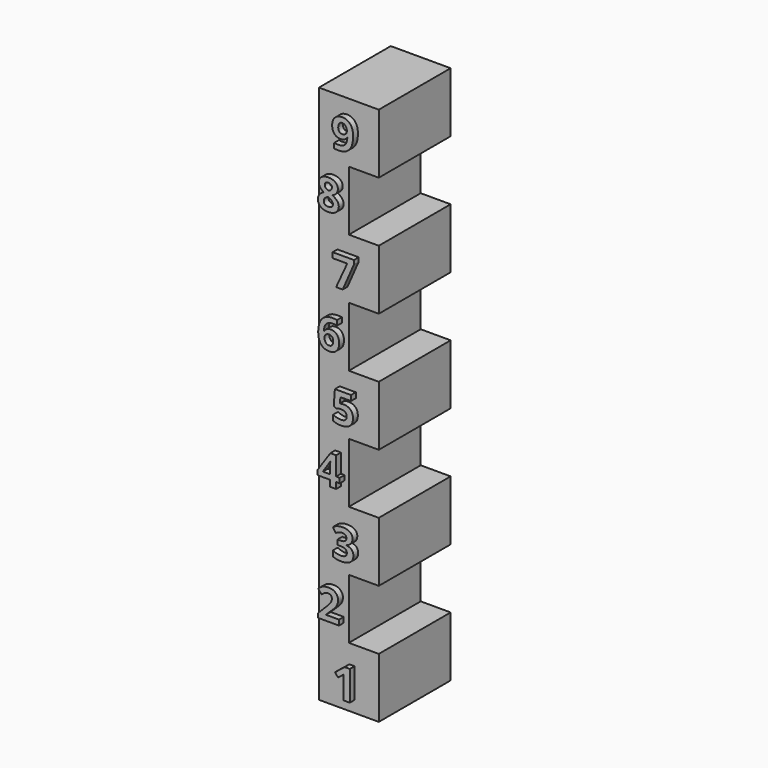
from build123d import *

# Parameters (mm, degrees)
F1_DEPTH     = 15
F2_TEXT_SIZE = 6.9444444444
F3_DEPTH     = 1
F4_TEXT_SIZE = 6.9444444444
F5_DEPTH     = 1


# Not quite as in the source:
# - Text() gives the source's letters only with a copy of the font that has no kerning and outlines rounded to 1/6400 em; it was checked with that copy


with BuildPart() as f1:
    # F0 (on Front) → F1 (new body)
    with BuildSketch(Plane.XZ):
        Polygon((17.6977999508, 53.6902362108), (17.6977999508, -36.3097637892), (22.6977999508, -36.3097637892), (27.6977999508, -36.3097637892), (27.6977999508, -26.3097637892), (22.6977999508, -26.3097637892), (22.6977999508, -16.3097637892), (27.6977999508, -16.3097637892), (27.6977999508, -6.3097637892), (22.6977999508, -6.3097637892), (22.6977999508, 3.6902362108), (27.6977999508, 3.6902362108), (27.6977999508, 13.6902362108), (22.6977999508, 13.6902362108), (22.6977999508, 23.6902362108), (27.6977999508, 23.6902362108), (27.6977999508, 33.6902362108), (22.6977999508, 33.6902362108), (22.6977999508, 43.6902362108), (27.6977999508, 43.6902362108), (27.6977999508, 53.6902362108), align=None)
    extrude(amount=F1_DEPTH)

    # F2 (on face) → F3 (join)
    with BuildSketch(Plane.XZ.offset(15)):
        with Locations((20.7831069488, -34.3956333771)):
            Text('1', F2_TEXT_SIZE, font='Open Sans', font_style=FontStyle.BOLD, text_align=(TextAlign.LEFT, TextAlign.BOTTOM))
        with Locations((18.1024699361, -23.6452650814)):
            Text('2', F2_TEXT_SIZE, font='Open Sans', font_style=FontStyle.BOLD, text_align=(TextAlign.LEFT, TextAlign.BOTTOM))
        with Locations((20.5617107408, -14.0193967335)):
            Text('3', F2_TEXT_SIZE, font='Open Sans', font_style=FontStyle.BOLD, text_align=(TextAlign.LEFT, TextAlign.BOTTOM))
        with Locations((18.1209300458, -3.7207709346)):
            Text('4', F2_TEXT_SIZE, font='Open Sans', font_style=FontStyle.BOLD, text_align=(TextAlign.LEFT, TextAlign.BOTTOM))
        with Locations((20.5431034747, 5.9468481503)):
            Text('5', F2_TEXT_SIZE, font='Open Sans', font_style=FontStyle.BOLD, text_align=(TextAlign.LEFT, TextAlign.BOTTOM))
        with Locations((18.136892487, 16.2113205343)):
            Text('6', F2_TEXT_SIZE, font='Open Sans', font_style=FontStyle.BOLD, text_align=(TextAlign.LEFT, TextAlign.BOTTOM))
        with Locations((20.6009032494, 25.9541989118)):
            Text('7', F2_TEXT_SIZE, font='Open Sans', font_style=FontStyle.BOLD, text_align=(TextAlign.LEFT, TextAlign.BOTTOM))
        with Locations((18.0933616431, 36.6414812207)):
            Text('8', F2_TEXT_SIZE, font='Open Sans', font_style=FontStyle.BOLD, text_align=(TextAlign.LEFT, TextAlign.BOTTOM))
        with Locations((20.4888266866, 46.2495227158)):
            Text('9', F2_TEXT_SIZE, font='Open Sans', font_style=FontStyle.BOLD, text_align=(TextAlign.LEFT, TextAlign.BOTTOM))
    extrude(amount=F3_DEPTH)

    # F4 (on face) → F5 (join)
    with BuildSketch(Plane(origin=(17.6977999508, 0, 0), x_dir=(0, -1, 0), z_dir=(-1, 0, 0))):
        with Locations((2.4972044713, 5.9488205612)):
            Text('C', F4_TEXT_SIZE, font='Open Sans', font_style=FontStyle.BOLD, text_align=(TextAlign.LEFT, TextAlign.BOTTOM))
    extrude(amount=F5_DEPTH)


solid = f1.part
